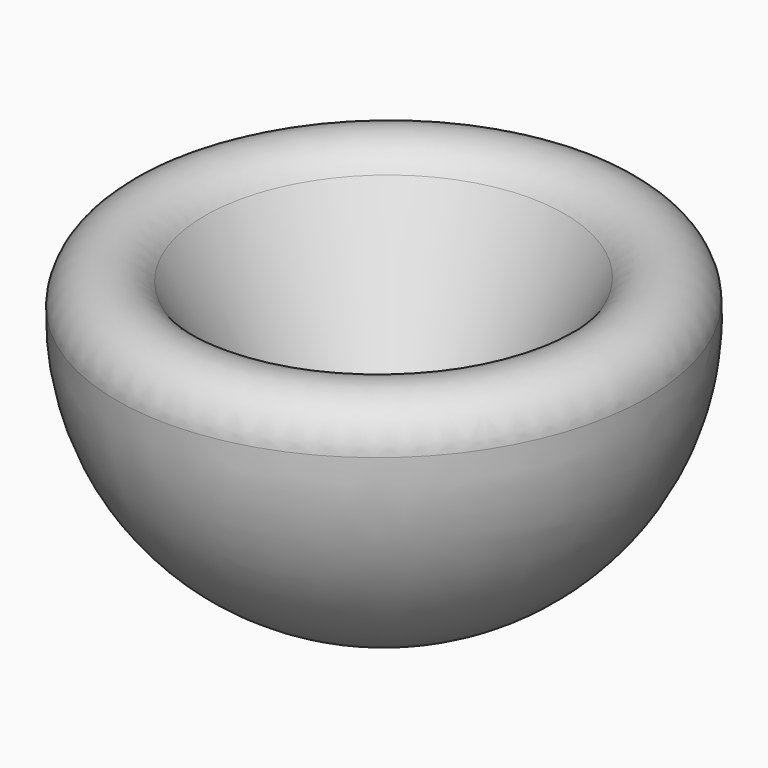
from build123d import *

# Parameters (mm, degrees)
F2_R = 5.08


with BuildPart() as f1:
    # F0 (on Front) → F1 (revolve)
    with BuildSketch(Plane.XZ):
        with BuildLine():
            ThreePointArc((0, -25.22482723), (24.331319664, -10.9412104356), (24.5950266565, 17.271646278))
            Line((24.5950266565, 17.271646278), (0, -25.22482723))
        make_face()
    revolve(axis=Axis((-1.1091685811, 0, 0.7882770151), (0.0129668674, 0, -0.9999159266)))

    # F2
    f2_edges = [f1.edges().sort_by_distance(p)[0] for p in [
        (-27.232159, 0, 16.599554),
    ]]
    fillet(f2_edges, radius=F2_R)


solid = f1.part
